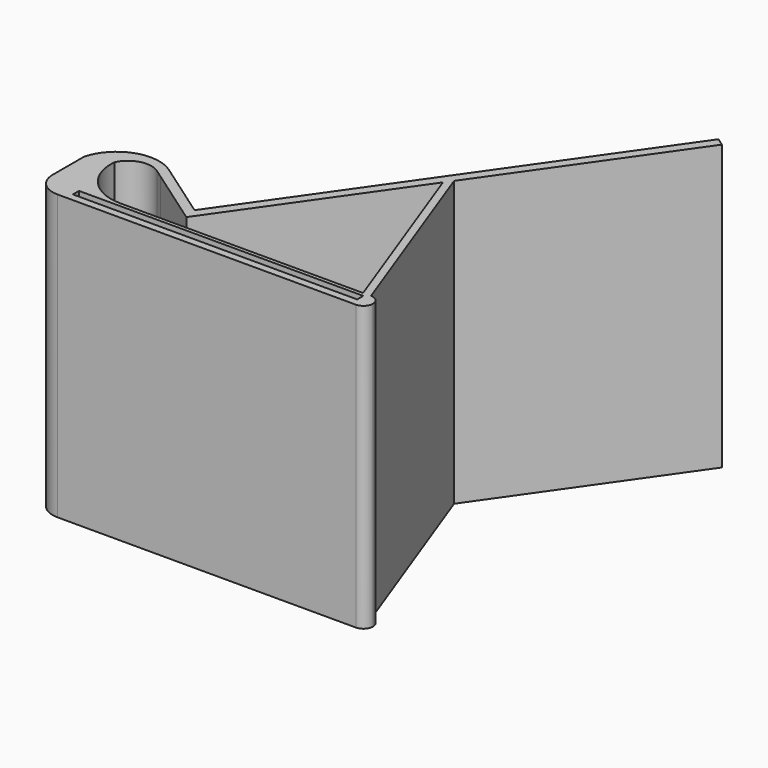
from build123d import *

# Parameters (mm, degrees)
F1_DEPTH    = 76.2
F2_W        = 76.2
F2_H        = 3.08
F3_DEPTH    = 71.12
F4_W        = 76.2
F4_H        = 2.54
F5_DEPTH    = 2.032
F6_T4_DEPTH = 76.2
F8_DEPTH    = 76.2


# Not quite as in the source:
# - a fillet or chamfer that OpenCascade refuses, or shapes differently, is made with other operations: its cross-section is extruded or revolved along the edge and cut away or added


with BuildPart() as f1:
    # F0 (on Top) → F1 (new body)
    with BuildSketch(Plane.XY):
        with BuildLine():
            Line((-71.12, 0), (-2.54, 0))
            ThreePointArc((-2.54, 0), (-0.7439487758, 0.7439487758), (0, 2.54))
            ThreePointArc((0, 2.54), (-0.7439487758, 4.3360512242), (-2.54, 5.08))
            Line((-2.54, 5.08), (-69.676465438, 5.08))
            ThreePointArc((-69.676465438, 5.08), (-79.0448551931, 9.2054286756), (-82.3268475088, 18.9015317486))
            ThreePointArc((-82.3268475088, 18.9015317486), (-78.2116767293, 22.3014792843), (-72.9571412523, 21.3611970334))
            Line((-72.9571412523, 21.3611970334), (-70.7962627974, 19.8481336501))
            Line((-70.7962627974, 19.8481336501), (-55.0490144099, 8.8217916231))
            Line((-55.0490144099, 8.8217916231), (11.9676564134, 104.5315164778))
            Line((11.9676564134, 104.5315164778), (9.8870102209, 105.9884006261))
            Line((9.8870102209, 105.9884006261), (-55.672776454, 12.3593219639))
            Line((-55.672776454, 12.3593219639), (-71.2776228977, 23.2859530764))
            ThreePointArc((-71.2776228977, 23.2859530764), (-81.747690686, 24.661984001), (-88.8767730732, 16.871479209))
            Line((-88.8767730732, 16.871479209), (-88.8912459344, 6.3587420222))
            ThreePointArc((-88.8912459344, 6.3587420222), (-87.0344697211, 1.8629637755), (-82.541251952, 0))
            Line((-82.541251952, 0), (-71.12, 0))
        make_face()
    extrude(amount=F1_DEPTH)

    # F2 (on face) → F3 (cut)
    with BuildSketch(Plane.XY.offset(76.2)):
        with Locations((-41.91, 2.54)):
            Rectangle(F2_W, F2_H)
    extrude(amount=-F3_DEPTH, mode=Mode.SUBTRACT)

    # F4 (on Front) → F5 (join)
    with BuildSketch(Plane.XZ):
        with Locations((-41.91, 74.93)):
            Rectangle(F4_W, F4_H)
    extrude(amount=-F5_DEPTH)

    # F6: chamfer of 2.54 on 1 edges, made by hand


with BuildPart() as f6_tool2:
    # F6_s3 → F6_t4 (new body)
    with BuildSketch(Plane.YZ.offset(-80.01)):
        Polygon((-0.508, 73.66), (2.032, 76.2), (2.032, 73.66), align=None)
    extrude(amount=F6_T4_DEPTH)

    split(bisect_by=Plane.XZ.offset(-1), keep=Keep.BOTTOM)


with BuildPart() as f1_1:
    add(f1.part)

    # F6_t1: cut F6_tool2
    add(f6_tool2.part, mode=Mode.SUBTRACT)

    # F7 (on face) → F8 (join)
    with BuildSketch(Plane.XY.offset(76.2)):
        Polygon((-4.6713010828, 5.08), (-2.54, 5.08), (-21.5406789982, 56.6766540504), (-22.9374096266, 54.6819159876), align=None)
    extrude(amount=-F8_DEPTH)


solid = f1_1.part
